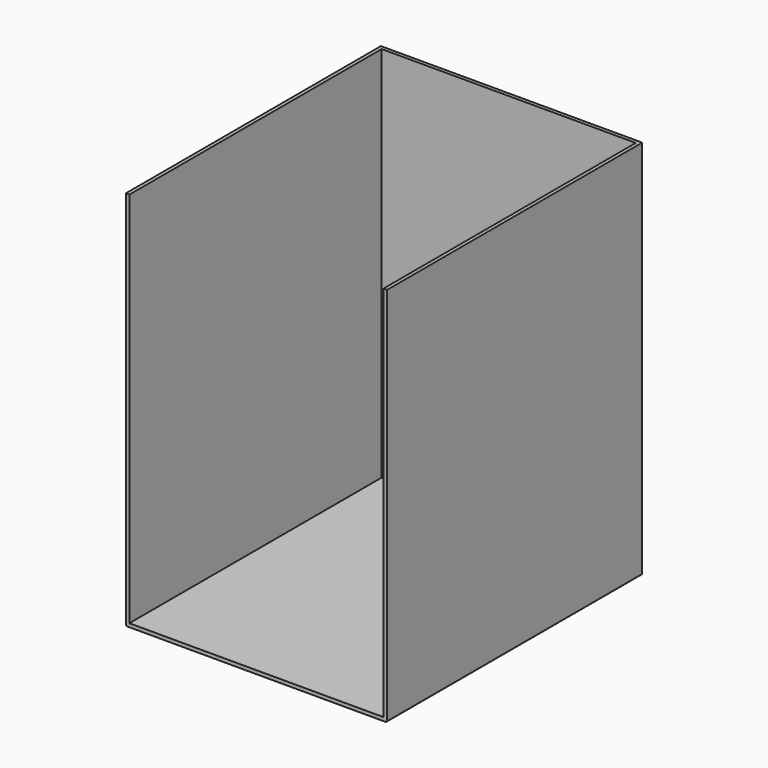
from build123d import *

# Parameters (mm, degrees)
F1_DEPTH = 426
F2_W     = 295
F2_H     = 360
F3_DEPTH = 4
F4_R     = 2


# Not quite as in the source:
# - a feature names something its author has since deleted; it is built from what else it names


with BuildPart() as f1:
    # F0 (on Top) → F1 (new body)
    with BuildSketch(Plane.XY):
        Polygon((-4, -360), (0, -360), (0, 0), (-295, 0), (-295, -360), (-291, -360), (-291, -4), (-4, -4), align=None)
    extrude(amount=F1_DEPTH)

    # F2 (on Top) → F3 (join)
    with BuildSketch(Plane.XY):
        with Locations((-147.5, -180)):
            Rectangle(F2_W, F2_H)
    extrude(amount=-F3_DEPTH)

    # F4
    f4_edges = [f1.edges().sort_by_distance(p)[0] for p in [
        (-295, -180, -4),
        (0, -180, -4),
    ]]
    fillet(f4_edges, radius=F4_R)


solid = f1.part
